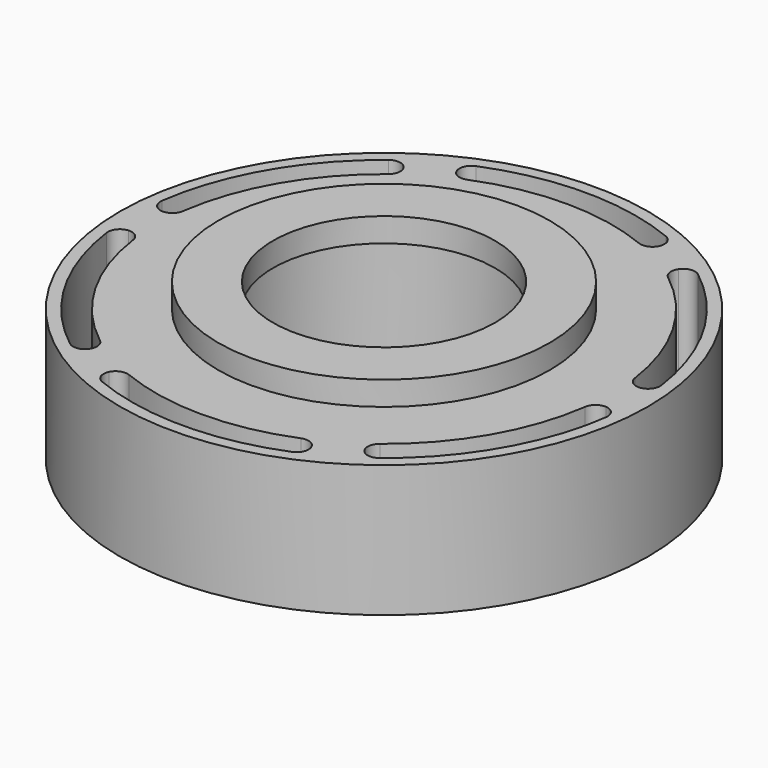
from build123d import *

# Parameters (mm, degrees)
F0_R            = 55.88
F0_R_2          = 27.432
F1_DEPTH        = 27.94
F2_R            = 35.052
F2_R_2          = 23.495
F3_DEPTH        = 5.08
F5_DEPTH        = 27.941
F5_COPIES_COUNT = 6
F6_R            = 2.53999


# Not quite as in the source:
# - a fillet or chamfer is up to 0.001 mm smaller than in the source, because OpenCascade refuses the exact size
# - a pattern or mirror of a feature is missing from the dataset's text; its kind, count and spacing are read off the source's solid


with BuildPart() as f1:
    # F0 (on Top) → F1 (new body)
    with BuildSketch(Plane.XY):
        Circle(F0_R)
        Circle(F0_R_2, mode=Mode.SUBTRACT)
    extrude(amount=F1_DEPTH)

    # F2 (on face) → F3 (join)
    with BuildSketch(Plane.XY.offset(27.94)):
        Circle(F2_R)
        Circle(F2_R_2, mode=Mode.SUBTRACT)
    extrude(amount=F3_DEPTH)

    # F4 (on face) → F5 (cut, through all)
    with BuildSketch(Plane.XY.offset(27.94)):
        with BuildLine():
            ThreePointArc((20.3955573116, -43.7384138024), (0, -48.26), (-20.3955573116, -43.7384138024))
            Line((-20.3955573116, -43.7384138024), (-22.5424580812, -48.3424573605))
            ThreePointArc((-22.5424580812, -48.3424573605), (0, -53.34), (22.5424580812, -48.3424573605))
            Line((22.5424580812, -48.3424573605), (20.3955573116, -43.7384138024))
        make_face()
    f5 = extrude(amount=-F5_DEPTH, mode=Mode.SUBTRACT)

    # F5_copies: F5 ×6 about axis
    f5_copies_axis = Axis((0, 0, 0), (0, 0, 1))
    for i in range(1, F5_COPIES_COUNT):
        add(f5.rotate(f5_copies_axis, i * 360 / F5_COPIES_COUNT), mode=Mode.SUBTRACT)

    # F6 (radius 2.54 in the source; OpenCascade refuses exactly that, so slightly less here)
    f6_edges = [f1.edges().sort_by_distance(p)[0] for p in [
        (-22.542458, -48.342457, 13.97),
        (-20.395557, -43.738414, 13.97),
        (22.542458, -48.342457, 13.97),
        (20.395557, -43.738414, 13.97),
        (-53.137025, -4.648887, 13.97),
        (-48.076356, -4.206136, 13.97),
        (-30.594567, -43.69357, 13.97),
        (-27.680799, -39.532278, 13.97),
        (30.594567, -43.69357, 13.97),
        (27.680799, -39.532278, 13.97),
        (48.076356, -4.206136, 13.97),
        (53.137025, -4.648887, 13.97),
        (-30.594567, 43.69357, 13.97),
        (-27.680799, 39.532278, 13.97),
        (-48.076356, 4.206136, 13.97),
        (-53.137025, 4.648887, 13.97),
        (22.542458, 48.342457, 13.97),
        (20.395557, 43.738414, 13.97),
        (-20.395557, 43.738414, 13.97),
        (-22.542458, 48.342457, 13.97),
        (53.137025, 4.648887, 13.97),
        (48.076356, 4.206136, 13.97),
        (27.680799, 39.532278, 13.97),
        (30.594567, 43.69357, 13.97),
    ]]
    fillet(f6_edges, radius=F6_R)


solid = f1.part
